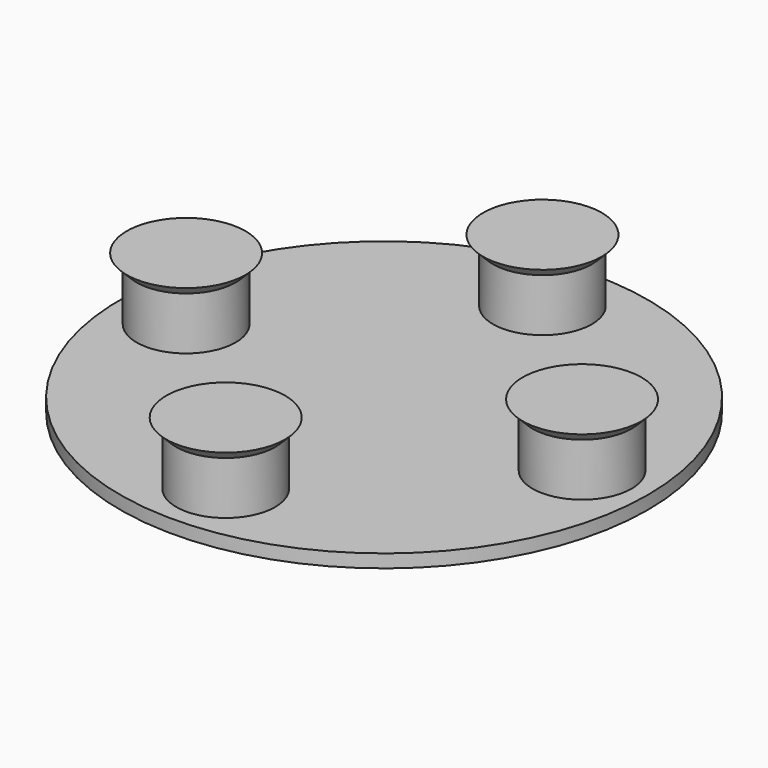
from build123d import *

# Parameters (mm, degrees)
F0_R     = 40
F0_R_2   = 7.5
F1_DEPTH = 2
F2_DEPTH = 10
F3_R     = 9
F3_R_2   = 7.5
F4_DEPTH = 1.5
F5_SIZE  = 1.49999


# Not quite as in the source:
# - a fillet or chamfer is up to 0.001 mm smaller than in the source, because OpenCascade refuses the exact size


with BuildPart() as f1:
    # F0 (on Top) → F1 (new body)
    with BuildSketch(Plane.XY):
        Circle(F0_R)
        with Locations((0, -30)):
            Circle(F0_R_2, mode=Mode.SUBTRACT)
        with Locations((-30, 0)):
            Circle(F0_R_2, mode=Mode.SUBTRACT)
        with Locations((30, 0)):
            Circle(F0_R_2, mode=Mode.SUBTRACT)
        with BuildLine():
            ThreePointArc((0, 22.5), (-5.3033008589, 35.3033008589), (7.5, 30))
            ThreePointArc((7.5, 30), (5.3033008589, 24.6966991411), (0, 22.5))
        make_face(mode=Mode.SUBTRACT)
    extrude(amount=F1_DEPTH)

    # F0 (on Top) → F2 (join)
    with BuildSketch(Plane.XY):
        with Locations((0, -30)):
            Circle(F0_R_2)
        with Locations((30, 0)):
            Circle(F0_R_2)
        with BuildLine():
            ThreePointArc((0, 22.5), (5.3033008589, 24.6966991411), (7.5, 30))
            ThreePointArc((7.5, 30), (-5.3033008589, 35.3033008589), (0, 22.5))
        make_face()
        with Locations((-30, 0)):
            Circle(F0_R_2)
    extrude(amount=F2_DEPTH)

    # F3 (on face) → F4 (join)
    with BuildSketch(Plane.XY.offset(10)):
        with Locations((-30, 0)):
            Circle(F3_R)
        with Locations((0, -30)):
            Circle(F3_R)
        with Locations((0, -30)):
            Circle(F3_R_2, mode=Mode.SUBTRACT)
        with Locations((0, -30)):
            Circle(F3_R_2)
        with Locations((30, 0)):
            Circle(F3_R)
        with Locations((0, 30)):
            Circle(F3_R)
    extrude(amount=F4_DEPTH)

    # F5 (size 1.5 in the source; OpenCascade refuses exactly that, so slightly less here)
    f5_edges = [f1.edges().sort_by_distance(p)[0] for p in [
        (-9, 30, 10),
        (-39, 0, 10),
        (-9, -30, 10),
        (21, 0, 10),
    ]]
    chamfer(f5_edges, length=F5_SIZE)


solid = f1.part
